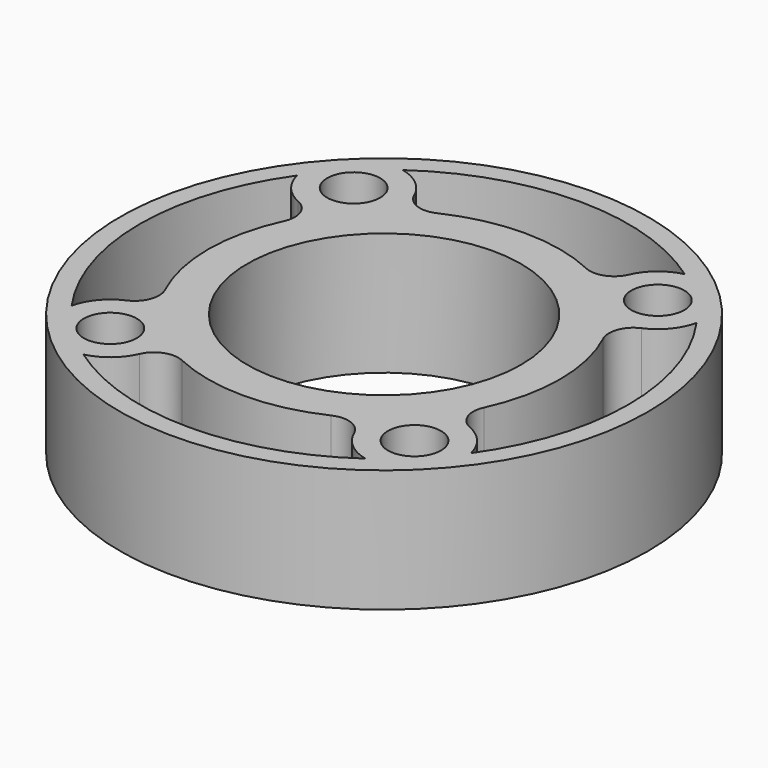
from build123d import *

# Parameters (mm, degrees)
F0_R            = 21.43125
F0_R_2          = 2.15265
F0_R_3          = 11.1125
F1_DEPTH        = 9.9568
F3_DEPTH        = 9.9568
F3_COPIES_COUNT = 4
F4_R            = 1.984375


# Not quite as in the source:
# - a pattern or mirror of a feature is missing from the dataset's text; its kind, count and spacing are read off the source's solid


with BuildPart() as f1:
    # F0 (on Top) → F1 (new body)
    with BuildSketch(Plane.XY):
        Circle(F0_R)
        with Locations((-12.3478521665, -12.3478521665)):
            Circle(F0_R_2, mode=Mode.SUBTRACT)
        with Locations((12.3478521665, -12.3478521665)):
            Circle(F0_R_2, mode=Mode.SUBTRACT)
        with Locations((-12.3478521665, 12.3478521665)):
            Circle(F0_R_2, mode=Mode.SUBTRACT)
        Circle(F0_R_3, mode=Mode.SUBTRACT)
        with Locations((12.3478521665, 12.3478521665)):
            Circle(F0_R_2, mode=Mode.SUBTRACT)
    extrude(amount=F1_DEPTH)

    # F2 (on face) → F3 (cut, through all)
    with BuildSketch(Plane.XY.offset(9.9568)):
        with BuildLine():
            ThreePointArc((8.4692641257, 11.5067033254), (8.9929440308, 14.4681276118), (11.4430257563, 16.212081162))
            ThreePointArc((11.4430257563, 16.212081162), (0, 19.84375), (-11.4430257563, 16.212081162))
            ThreePointArc((-11.4430257563, 16.212081162), (-8.9929440308, 14.4681276118), (-8.4692641257, 11.5067033254))
            ThreePointArc((-8.4692641257, 11.5067033254), (0, 14.2875), (8.4692641257, 11.5067033254))
        make_face()
    f3 = extrude(amount=-F3_DEPTH, mode=Mode.SUBTRACT)

    # F3_copies: F3 ×4 about axis
    f3_copies_axis = Axis((0, 0, 0), (0, 0, 1))
    for i in range(1, F3_COPIES_COUNT):
        add(f3.rotate(f3_copies_axis, i * 360 / F3_COPIES_COUNT), mode=Mode.SUBTRACT)

    # F4
    f4_edges = [f1.edges().sort_by_distance(p)[0] for p in [
        (8.469264, 11.506703, 4.9784),
        (-8.469264, 11.506703, 4.9784),
        (8.469264, -11.506703, 4.9784),
        (-8.469264, -11.506703, 4.9784),
        (11.506703, 8.469264, 4.9784),
        (11.506703, -8.469264, 4.9784),
        (-11.506703, -8.469264, 4.9784),
        (-11.506703, 8.469264, 4.9784),
    ]]
    fillet(f4_edges, radius=F4_R)


solid = f1.part
